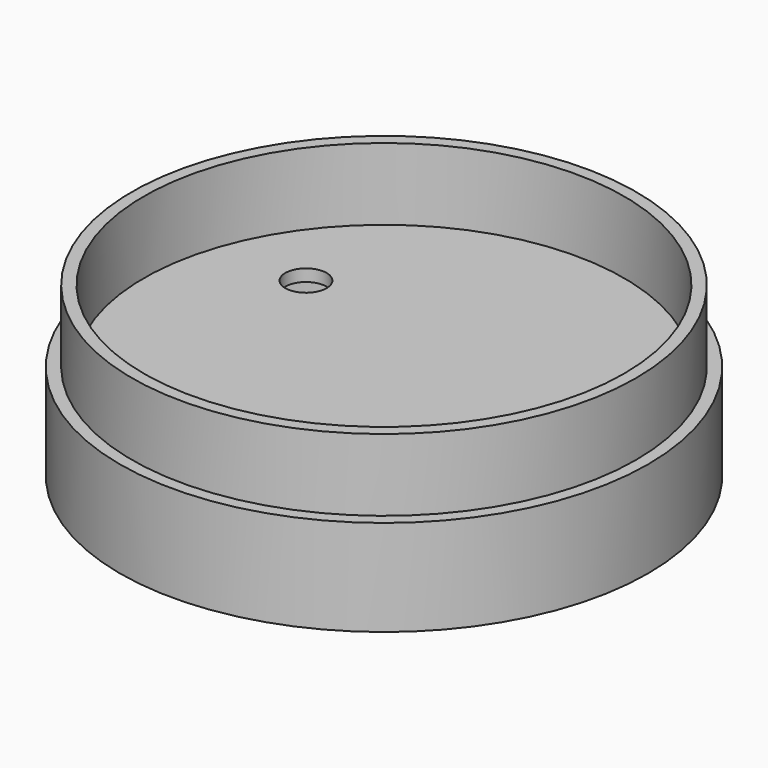
from build123d import *

# Parameters (mm, degrees)
F3_DEPTH = 5
F4_R     = 2.58
F5_DEPTH = 25


# Not quite as in the source:
# - ends of sketch curves that miss each other by under 0.0002 mm in the source are joined


with BuildPart() as f1:
    # F0 (on Front) → F1 (revolve)
    with BuildSketch(Plane.XZ):
        Polygon((30, 0), (0, 0), (0, -1.5), (30, -1.5), (30, -12), (33, -12), (33, 0), (31.5, 0), (31.5, 9), (30, 9), align=None)
    revolve(axis=Axis((0, 0, -0.75), (0, 0, 1)))

    # F2 (on face) → F3 (cut)
    with BuildSketch(Plane(origin=(0, 0, -12), x_dir=(1, 0, 0), z_dir=(0, 0, -1))):
        with BuildLine():
            Line((-5, 31.030934304), (-5, 29.5803989155))
            ThreePointArc((-5, 29.5803989155), (0, 30), (5, 29.5803989155))
            Line((5, 29.5803989155), (5, 31.0276464719))
            ThreePointArc((5, 31.0276464719), (0.0001313019, 31.4286473296), (-5, 31.030934304))
        make_face()
        with BuildLine():
            Line((-29.5821256825, 4.9897735526), (-31.1022785476, 4.9897735526))
            ThreePointArc((-31.1022785476, 4.9897735526), (-31.5, 0), (-31.1022852718, -4.9897746313))
            Line((-31.1022852718, -4.9897746313), (-29.5821255005, -4.9897746313))
            ThreePointArc((-29.5821255005, -4.9897746313), (-30, -5.47e-07), (-29.5821256825, 4.9897735526))
        make_face()
        with BuildLine():
            ThreePointArc((5, -29.5803989155), (0, -30), (-5, -29.5803989155))
            Line((-5, -29.5803989155), (-5, -31.1736362396))
            ThreePointArc((-5, -31.1736362396), (0.0001313019, -31.5713492653), (5, -31.1703484075))
            Line((5, -31.1703484075), (5, -29.5803989155))
        make_face()
        with BuildLine():
            Line((31.1022785476, 4.9897735526), (29.5821256825, 4.9897735526))
            ThreePointArc((29.5821256825, 4.9897735526), (29.8953488897, 2.5036203312), (30, 0))
            ThreePointArc((30, 0), (29.8953488441, -2.5036208763), (29.5821255005, -4.9897746313))
            Line((29.5821255005, -4.9897746313), (31.1022852718, -4.9897746313))
            ThreePointArc((31.1022852718, -4.9897746313), (31.5, 0), (31.1022785476, 4.9897735526))
        make_face()
    extrude(amount=-F3_DEPTH, mode=Mode.SUBTRACT)

    # F4 (on face) → F5 (cut)
    with BuildSketch(Plane.XY.offset(9)):
        with Locations((-17.3232257366, 9.4686336815)):
            Circle(F4_R)
    extrude(amount=-F5_DEPTH, mode=Mode.SUBTRACT)


solid = f1.part
